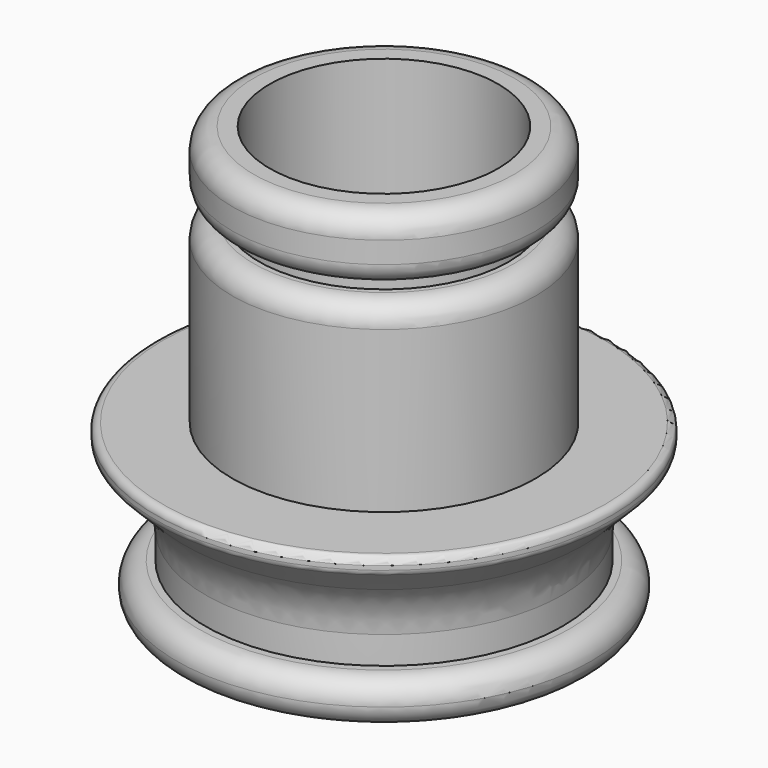
from build123d import *

# Parameters (mm, degrees)
F0_R        = 14.5
F1_DEPTH    = 3
F3_R        = 12.5
F4_DEPTH    = 3.5
F6_R        = 16
F7_DEPTH    = 5
F8_R        = 1.49999
F9_S5_R     = 12.5
F9_T6_DEPTH = 24
F10_R       = 5
F11_R       = 0.5
F13_R       = 10.625
F14_DEPTH   = 12.75
F16_R       = 8.75
F17_DEPTH   = 1
F19_R       = 10.625
F20_DEPTH   = 4.5
F21_R       = 1.5
F23_R       = 8
F24_DEPTH   = 25


# Not quite as in the source:
# - a fillet or chamfer that OpenCascade refuses, or shapes differently, is made with other operations: its cross-section is extruded or revolved along the edge and cut away or added
# - a fillet or chamfer is up to 0.001 mm smaller than in the source, because OpenCascade refuses the exact size


with BuildPart() as f1:
    # F0 (on Top) → F1 (new body)
    with BuildSketch(Plane.XY):
        Circle(F0_R)
    extrude(amount=F1_DEPTH)

    # F3 (on offset) → F4 (join)
    with BuildSketch(Plane.XY.offset(3)):
        Circle(F3_R)
    extrude(amount=F4_DEPTH)

    # F6 (on offset) → F7 (join)
    with BuildSketch(Plane.XY.offset(6.5)):
        Circle(F6_R)
    extrude(amount=F7_DEPTH)

    # F8 (radius 1.5 in the source; OpenCascade refuses exactly that, so slightly less here)
    f8_edges = [f1.edges().sort_by_distance(p)[0] for p in [
        (-14.5, 0, 0),
        (-14.5, 0, 3),
    ]]
    fillet(f8_edges, radius=F8_R)

    # F9: chamfer of 4 on 1 edges, made by hand


with BuildPart() as f9_tool2:
    # F9_s3 → F9_t4 (revolve)
    with BuildSketch(Plane.XZ):
        Polygon((12, 6.5), (16, 10.5), (16, 6.5), align=None)
    revolve(axis=Axis((0, 0, 6.5), (0, 0, 1)))

    # F9_s5 → F9_t6 (cut, symmetric)
    with BuildSketch(Plane.XY.offset(8.5)):
        Circle(F9_S5_R)
    extrude(amount=F9_T6_DEPTH, both=True, mode=Mode.SUBTRACT)


with BuildPart() as f1_1:
    add(f1.part)

    # F9_t1: cut F9_tool2
    add(f9_tool2.part, mode=Mode.SUBTRACT)

    # F10
    f10_edges = [f1_1.edges().sort_by_distance(p)[0] for p in [
        (-12.5, 0, 7),
    ]]
    fillet(f10_edges, radius=F10_R)

    # F11
    f11_edges = [f1_1.edges().sort_by_distance(p)[0] for p in [
        (-16, 0, 10.5),
        (-16, 0, 11.5),
    ]]
    fillet(f11_edges, radius=F11_R)

    # F13 (on offset) → F14 (join)
    with BuildSketch(Plane.XY.offset(11.5)):
        Circle(F13_R)
    extrude(amount=F14_DEPTH)

    # F16 (on offset) → F17 (join)
    with BuildSketch(Plane.XY.offset(24.25)):
        Circle(F16_R)
    extrude(amount=F17_DEPTH)

    # F19 (on offset) → F20 (join)
    with BuildSketch(Plane.XY.offset(25.25)):
        Circle(F19_R)
    extrude(amount=F20_DEPTH)

    # F21
    f21_edges = [f1_1.edges().sort_by_distance(p)[0] for p in [
        (-10.625, 0, 24.25),
        (-10.625, 0, 25.25),
        (-10.625, 0, 29.75),
    ]]
    fillet(f21_edges, radius=F21_R)

    # F23 (on offset) → F24 (cut)
    with BuildSketch(Plane.XY.offset(29.75)):
        Circle(F23_R)
    extrude(amount=-F24_DEPTH, mode=Mode.SUBTRACT)


solid = f1_1.part
